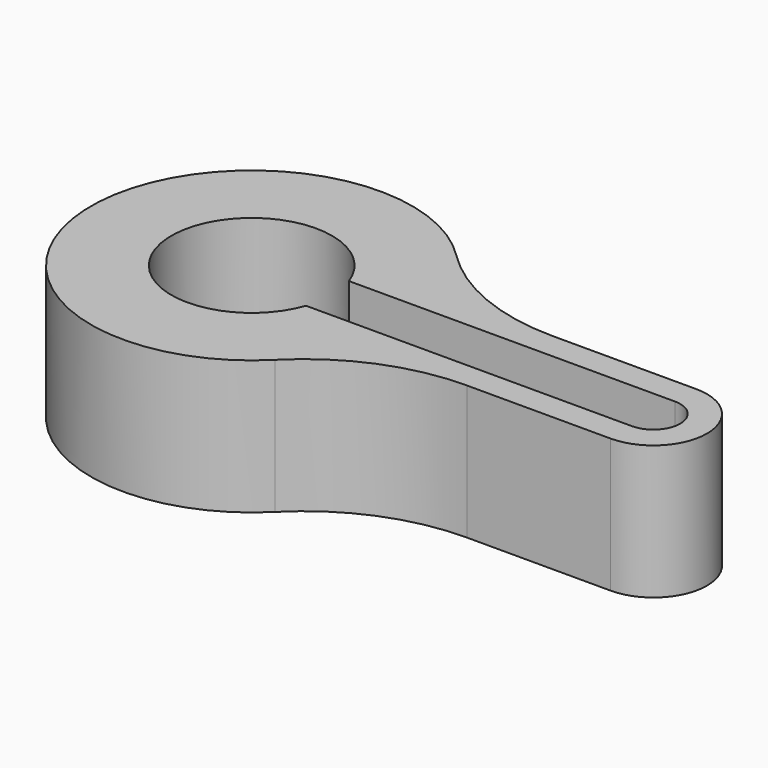
from build123d import *

# Parameters (mm, degrees)
F1_DEPTH = 25


# Not quite as in the source:
# - ends of sketch curves that miss each other by under 0.0002 mm in the source are joined


with BuildPart() as f1:
    # F0 (on Top) → F1 (new body)
    with BuildSketch(Plane.XY):
        with BuildLine():
            ThreePointArc((48.1663785379, 9.9999997765), (33.5940436684, 12.9051702933), (21.2498728844, 21.1764704896))
            ThreePointArc((21.2498728844, 21.1764704896), (-30, 6.96e-08), (21.2498727861, -21.1764705882))
            ThreePointArc((21.2498727861, -21.1764705882), (33.5940435271, -12.9051704831), (48.1663783152, -10))
            Line((48.1663783152, -10), (75, -10))
            ThreePointArc((75, -10), (84.9999997765, 0), (75, 9.9999997765))
            Line((75, 9.9999997765), (48.1663785379, 9.9999997765))
        make_face()
        with BuildLine():
            ThreePointArc((14.1421356237, -5), (-15, 0), (14.1421356237, 5))
            Line((14.1421356237, 5), (75, 5))
            ThreePointArc((75, 5), (80, 0), (75, -5))
            Line((75, -5), (14.1421356237, -5))
        make_face(mode=Mode.SUBTRACT)
    extrude(amount=F1_DEPTH)


solid = f1.part
